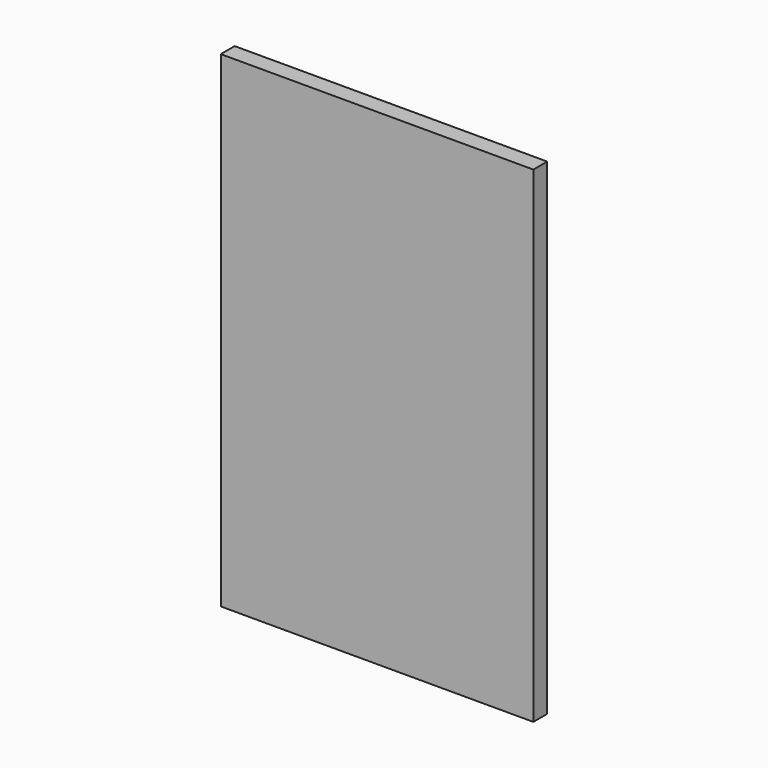
from build123d import *

# Parameters (mm, degrees)
F0_W     = 57.15
F0_H     = 88.9
F1_DEPTH = 3.175


# Not quite as in the source:
# - a length typed as a fraction of an inch, garbled in the dataset ("3 / 203.2 mm" for 3/8 in), is restored


with BuildPart() as f1:
    # F0 (on Front) → F1 (new body)
    with BuildSketch(Plane.XZ):
        with Locations((1.3294197339, 0)):
            Rectangle(F0_W, F0_H)
    extrude(amount=F1_DEPTH)


solid = f1.part
